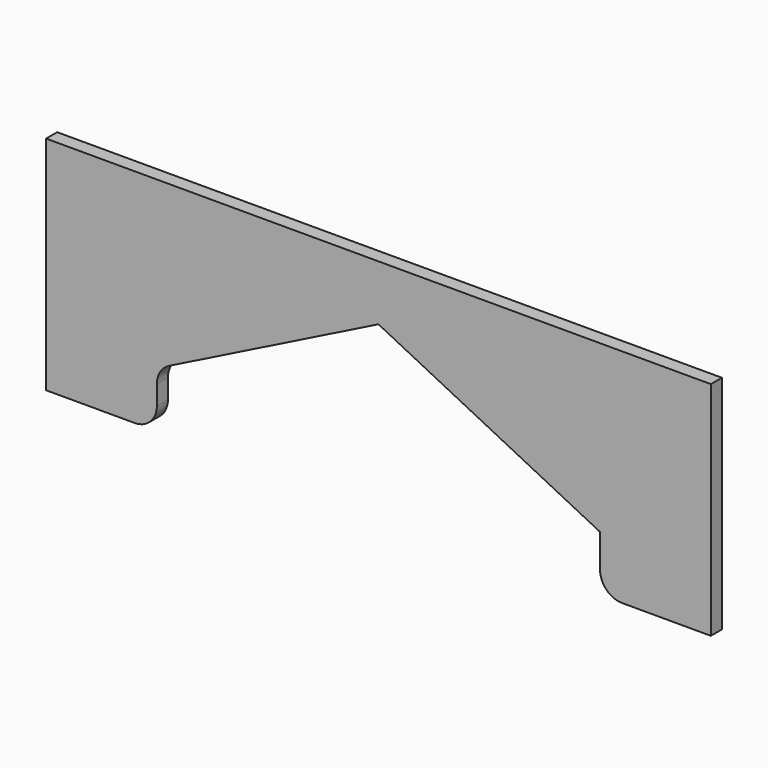
from build123d import *

# Parameters (mm, degrees)
F1_DEPTH = 3.175
F2_R     = 5.08
F3_R     = 5.08


# Not quite as in the source:
# - a feature names something its author has since deleted; it is built from what else it names


with BuildPart() as f1:
    # F0 (on Front) → F1 (new body)
    with BuildSketch(Plane.XZ):
        Polygon((45.1797973156, 19.05), (-107.2202026844, 19.05), (-107.2202026844, -31.75), (-81.8202026844, -31.75), (-81.8202026844, -19.05), (-31.0202026844, 6.35), (19.7797973156, -19.05), (19.7797973156, -31.75), (45.1797973156, -31.75), (45.1797973156, -6.35), align=None)
    extrude(amount=F1_DEPTH)

    # F2
    f2_edges = [f1.edges().sort_by_distance(p)[0] for p in [
        (-81.820203, -1.5875, -19.05),
    ]]
    fillet(f2_edges, radius=F2_R)

    # F3
    f3_edges = [f1.edges().sort_by_distance(p)[0] for p in [
        (-81.820203, -1.5875, -31.75),
        (19.779797, -1.5875, -31.75),
    ]]
    fillet(f3_edges, radius=F3_R)


solid = f1.part
